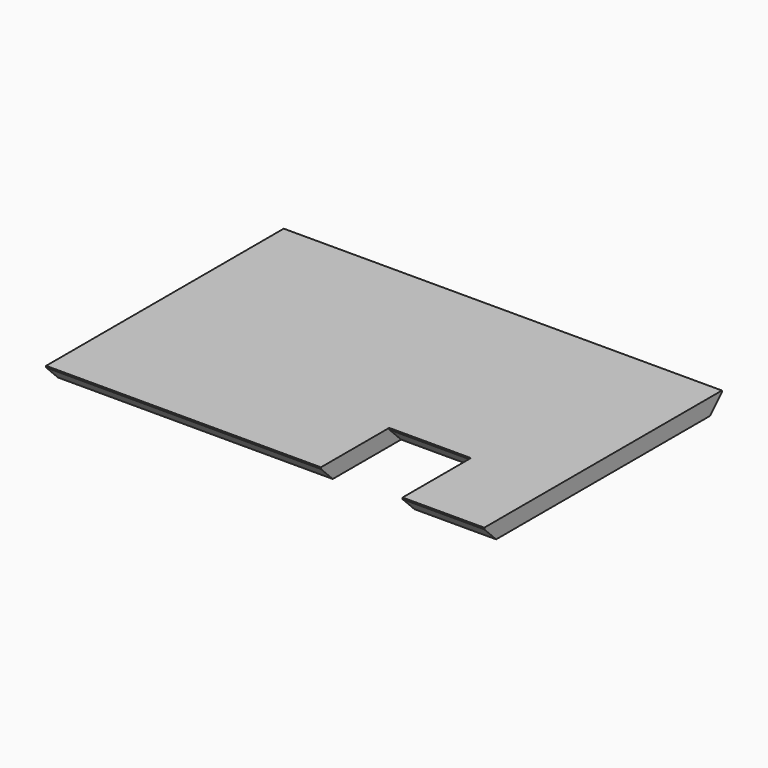
from build123d import *

# Parameters (mm, degrees)
F1_DEPTH = 2.2
F2_SIZE  = 2
F3_SIZE  = 2


with BuildPart() as f1:
    # F0 (on Top) → F1 (new body)
    with BuildSketch(Plane.XY):
        Polygon((-0.1190041415, 38.1740419386), (-59.1190041415, 38.1740419386), (-59.1190041415, -1.8259580614), (-22.1190041415, -1.8259580614), (-22.1190041415, 9.6740419386), (-11.1190041415, 9.6740419386), (-11.1190041415, -1.8259580614), (-0.1190041415, -1.8259580614), align=None)
    extrude(amount=F1_DEPTH)

    # F2
    f2_edges = [f1.edges().sort_by_distance(p)[0] for p in [
        (-29.619004, 38.174042, 0),
        (-40.619004, -1.825958, 0),
    ]]
    chamfer(f2_edges, length=F2_SIZE)

    # F3
    f3_edges = [f1.edges().sort_by_distance(p)[0] for p in [
        (-16.619004, 9.674042, 0),
        (-5.619004, -1.825958, 0),
    ]]
    chamfer(f3_edges, length=F3_SIZE)


solid = f1.part
